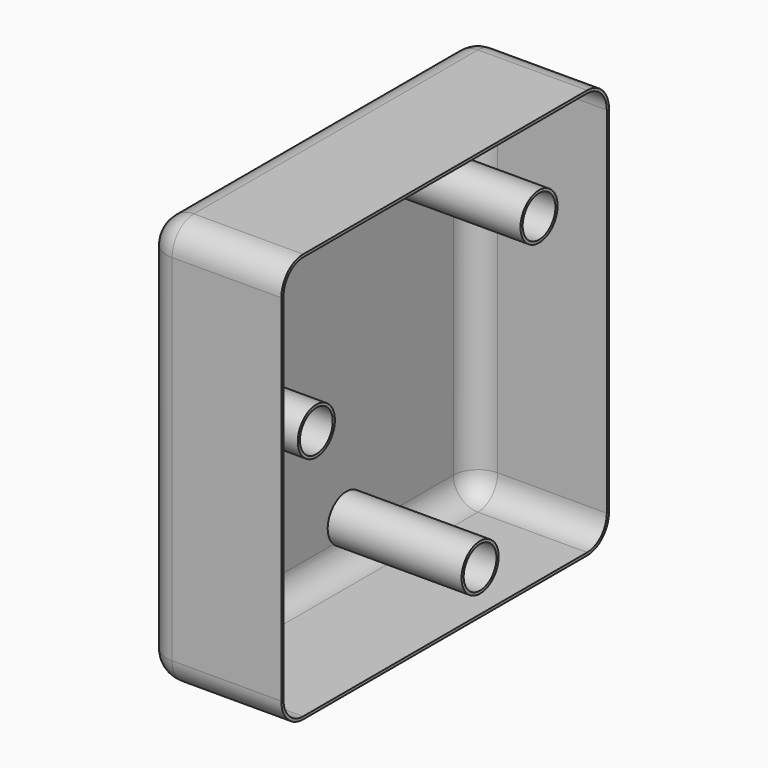
from build123d import *

# Parameters (mm, degrees)
F0_W         = 25.4
F0_H         = 76.2
F1_DEPTH     = 38.1
F3_D         = 7.62
F4_T1_DEPTH  = 66.04
F4_T3_DEPTH  = 66.04
F4_T5_DEPTH  = 33.02
F4_S9_W      = 5.08
F4_S9_H      = 5.08
F4_T10_DEPTH = 5.08
F4_S15_W     = 5.08
F4_S15_H     = 5.08
F4_T16_DEPTH = 5.08
F4_S21_W     = 5.08
F4_S21_H     = 5.08
F4_T22_DEPTH = 5.08
F4_S27_W     = 5.08
F4_S27_H     = 5.08
F4_T28_DEPTH = 5.08
F5_T         = -0.508


# Not quite as in the source:
# - a fillet or chamfer that OpenCascade refuses, or shapes differently, is made with other operations: its cross-section is extruded or revolved along the edge and cut away or added


with BuildPart() as f1:
    # F0 (on Front) → F1 (new body, symmetric)
    with BuildSketch(Plane.XZ):
        Rectangle(F0_W, F0_H)
    extrude(amount=F1_DEPTH, both=True)

    # F3 (through all)
    with Locations(Plane(origin=(-12.7, 0, 0), x_dir=(0, -1, 0), z_dir=(-1, 0, 0))):
        with Locations((29.9560025906, 7.917207202), (-21.8345038593, 21.9840556383), (-8.1214987313, -29.9012628403)):
            Hole(F3_D / 2)

    # F4: fillet of radius 5.08 on 8 edges, made by hand

    # F4_s2 → F4_t1 (cut)
    with BuildSketch(Plane.XZ.offset(-33.02)):
        with BuildLine():
            ThreePointArc((-7.62, 38.1), (-11.2121024484, 36.6121024484), (-12.7, 33.02))
            Line((-12.7, 33.02), (-12.7, 38.1))
            Line((-12.7, 38.1), (-7.62, 38.1))
        make_face()
        with BuildLine():
            ThreePointArc((-7.62, -38.1), (-11.2121024484, -36.6121024484), (-12.7, -33.02))
            Line((-12.7, -33.02), (-12.7, -38.1))
            Line((-12.7, -38.1), (-7.62, -38.1))
        make_face()
    extrude(amount=F4_T1_DEPTH, mode=Mode.SUBTRACT)

    # F4_s4 → F4_t3 (cut)
    with BuildSketch(Plane.XY.offset(-33.02)):
        with BuildLine():
            ThreePointArc((-7.62, 38.1), (-11.2121024484, 36.6121024484), (-12.7, 33.02))
            Line((-12.7, 33.02), (-12.7, 38.1))
            Line((-12.7, 38.1), (-7.62, 38.1))
        make_face()
        with BuildLine():
            ThreePointArc((-7.62, -38.1), (-11.2121024484, -36.6121024484), (-12.7, -33.02))
            Line((-12.7, -33.02), (-12.7, -38.1))
            Line((-12.7, -38.1), (-7.62, -38.1))
        make_face()
    extrude(amount=F4_T3_DEPTH, mode=Mode.SUBTRACT)

    # F4_s6 → F4_t5 (cut)
    with BuildSketch(Plane.YZ.offset(-7.62)):
        with BuildLine():
            ThreePointArc((38.1, 33.02), (36.6121024484, 36.6121024484), (33.02, 38.1))
            Line((33.02, 38.1), (38.1, 38.1))
            Line((38.1, 38.1), (38.1, 33.02))
        make_face()
        with BuildLine():
            ThreePointArc((38.1, -33.02), (36.6121024484, -36.6121024484), (33.02, -38.1))
            Line((33.02, -38.1), (38.1, -38.1))
            Line((38.1, -38.1), (38.1, -33.02))
        make_face()
        with BuildLine():
            ThreePointArc((-33.02, 38.1), (-36.6121024484, 36.6121024484), (-38.1, 33.02))
            Line((-38.1, 33.02), (-38.1, 38.1))
            Line((-38.1, 38.1), (-33.02, 38.1))
        make_face()
        with BuildLine():
            ThreePointArc((-33.02, -38.1), (-36.6121024484, -36.6121024484), (-38.1, -33.02))
            Line((-38.1, -33.02), (-38.1, -38.1))
            Line((-38.1, -38.1), (-33.02, -38.1))
        make_face()
    extrude(amount=F4_T5_DEPTH, mode=Mode.SUBTRACT)


with BuildPart() as f4_tool8:
    # F4_s9 → F4_t10 (new body)
    with BuildSketch(Plane.YZ.offset(-7.62)):
        with Locations((35.56, 35.56)):
            Rectangle(F4_S9_W, F4_S9_H)
    extrude(amount=-F4_T10_DEPTH)

    # F4_s11 → F4_t12 (revolve, cut)
    with BuildSketch(Plane(origin=(-7.62, 33.02, 33.02), x_dir=(0, -0.7071067812, -0.7071067812), z_dir=(0, 0.7071067812, -0.7071067812))):
        with BuildLine():
            ThreePointArc((0, -5.08), (5.08, 0), (0, 5.08))
            Line((0, 5.08), (0, -5.08))
        make_face()
    revolve(axis=Axis((-7.62, 33.02, 33.02), (-1, 0, 0)), mode=Mode.SUBTRACT)


with BuildPart() as f1_1:
    add(f1.part)

    # F4_t7: cut F4_tool8
    add(f4_tool8.part, mode=Mode.SUBTRACT)


with BuildPart() as f4_tool14:
    # F4_s15 → F4_t16 (new body)
    with BuildSketch(Plane.YZ.offset(-7.62)):
        with Locations((-35.56, 35.56)):
            Rectangle(F4_S15_W, F4_S15_H)
    extrude(amount=-F4_T16_DEPTH)

    # F4_s17 → F4_t18 (revolve, cut)
    with BuildSketch(Plane(origin=(-7.62, -33.02, 33.02), x_dir=(0, 0.7071067812, -0.7071067812), z_dir=(0, 0.7071067812, 0.7071067812))):
        with BuildLine():
            ThreePointArc((0, -5.08), (5.08, 0), (0, 5.08))
            Line((0, 5.08), (0, -5.08))
        make_face()
    revolve(axis=Axis((-7.62, -33.02, 33.02), (-1, 0, 0)), mode=Mode.SUBTRACT)


with BuildPart() as f1_2:
    add(f1_1.part)

    # F4_t13: cut F4_tool14
    add(f4_tool14.part, mode=Mode.SUBTRACT)


with BuildPart() as f4_tool20:
    # F4_s21 → F4_t22 (new body)
    with BuildSketch(Plane.YZ.offset(-7.62)):
        with Locations((35.56, -35.56)):
            Rectangle(F4_S21_W, F4_S21_H)
    extrude(amount=-F4_T22_DEPTH)

    # F4_s23 → F4_t24 (revolve, cut)
    with BuildSketch(Plane(origin=(-7.62, 33.02, -33.02), x_dir=(0, -0.7071067812, 0.7071067812), z_dir=(0, -0.7071067812, -0.7071067812))):
        with BuildLine():
            ThreePointArc((0, -5.08), (5.08, 0), (0, 5.08))
            Line((0, 5.08), (0, -5.08))
        make_face()
    revolve(axis=Axis((-7.62, 33.02, -33.02), (-1, 0, 0)), mode=Mode.SUBTRACT)


with BuildPart() as f1_3:
    add(f1_2.part)

    # F4_t19: cut F4_tool20
    add(f4_tool20.part, mode=Mode.SUBTRACT)


with BuildPart() as f4_tool26:
    # F4_s27 → F4_t28 (new body)
    with BuildSketch(Plane.YZ.offset(-7.62)):
        with Locations((-35.56, -35.56)):
            Rectangle(F4_S27_W, F4_S27_H)
    extrude(amount=-F4_T28_DEPTH)

    # F4_s29 → F4_t30 (revolve, cut)
    with BuildSketch(Plane(origin=(-7.62, -33.02, -33.02), x_dir=(0, 0.7071067812, 0.7071067812), z_dir=(0, -0.7071067812, 0.7071067812))):
        with BuildLine():
            ThreePointArc((0, -5.08), (5.08, 0), (0, 5.08))
            Line((0, 5.08), (0, -5.08))
        make_face()
    revolve(axis=Axis((-7.62, -33.02, -33.02), (-1, 0, 0)), mode=Mode.SUBTRACT)


with BuildPart() as f1_4:
    add(f1_3.part)

    # F4_t25: cut F4_tool26
    add(f4_tool26.part, mode=Mode.SUBTRACT)

    # F5
    f5_openings = [f1_4.faces().sort_by_distance(p)[0] for p in [
        (12.7, 0, 0),
    ]]
    offset(amount=F5_T, openings=f5_openings)


solid = f1_4.part
